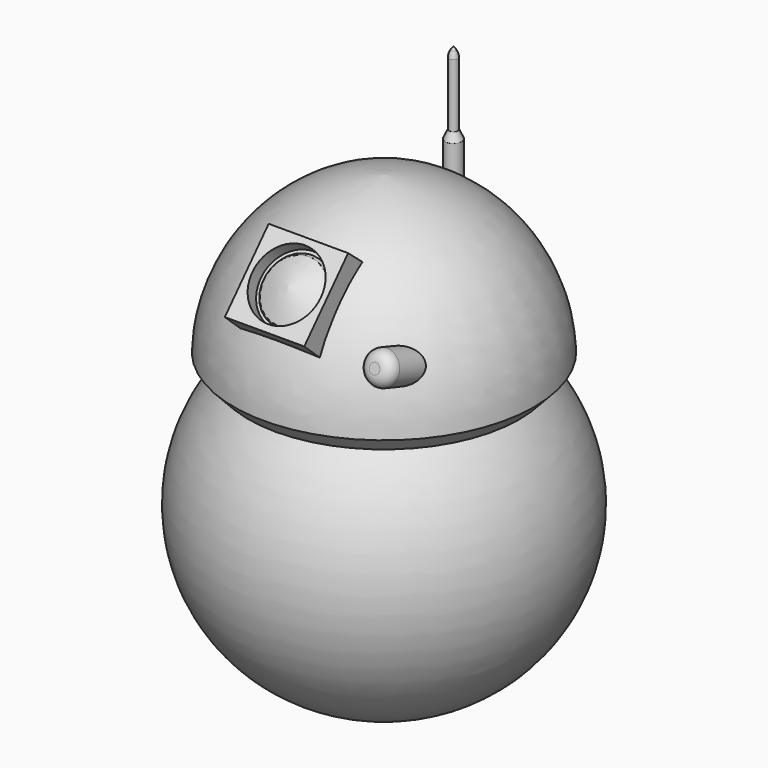
from build123d import *

# Parameters (mm, degrees)
F7_DEPTH = 18.288
F8_R     = 15.7921684899
F9_DEPTH = 6.604
F15_R    = 5.08
F16_R    = 5.08


with BuildPart() as f1:
    # F0 (on Front) → F1 (revolve)
    with BuildSketch(Plane.XZ):
        with BuildLine():
            Line((0, 77.0203024149), (0, -77.3050412536))
            ThreePointArc((0, -77.3050412536), (79.8093785121, -0.1423694193), (0, 77.0203024149))
        make_face()
    revolve(axis=Axis((0, 0, -0.1423694193), (0, 0, 1)))


with BuildPart() as f3:
    # F2 (on Front) → F3 (revolve)
    with BuildSketch(Plane.XZ):
        with BuildLine():
            Line((-69.1199526191, 61.6020485759), (-62.3490922153, 54.3798021972))
            ThreePointArc((-62.3490922153, 54.3798021972), (-33.4424698857, 72.8711770856), (0, 80.5604532361))
            Line((0, 80.5604532361), (0, 133.3731412888))
            ThreePointArc((0, 133.3731412888), (-48.2298855063, 110.6525536959), (-69.1199526191, 61.6020485759))
        make_face()
    revolve(axis=Axis((0, 0, 106.9667972624), (0, 0, 1)))


with BuildPart() as f5:
    # F4 (on Right) → F5 (revolve)
    with BuildSketch(Plane.YZ):
        with BuildLine():
            Line((-37.6473630313, 117.5783574581), (-43.1099124253, 117.5783574581))
            add(Edge.make_bspline(
                [(-43.1099124253, 117.5783574581), (-45.6695191469, 116.4036462387), (-50.3685346331, 114.2470703222), (-54.3983321793, 110.6990953442), (-55.3145445883, 110.0981011987)],
                knots=[0, 0, 0, 0, 0.4632741416, 0.8504948621, 0.8504948621, 0.8504948621, 0.8504948621], degree=3))
            Line((-55.3145445883, 110.0981011987), (-49.0153767169, 104.5863330364))
            Line((-49.0153767169, 104.5863330364), (-37.6473630313, 117.5783574581))
        make_face()
    revolve(axis=Axis((0, -52.1649606526, 107.3422171175), (0, 0.7525769153, -0.6585043558)))


with BuildPart() as f7:
    # F6 (on Right) → F7 (new body, symmetric)
    with BuildSketch(Plane.YZ):
        Polygon((-59.645216912, 89.2321169376), (-34.054864198, 117.1846613288), (-43.5066700909, 125.1279643094), (-68.7435230148, 97.561550531), align=None)
    extrude(amount=F7_DEPTH, both=True)


with BuildPart() as f9_tool:
    # F8 (on face) → F9 (new body)
    with BuildSketch(Plane(origin=(0, -85.9899317235, 78.7231620803), x_dir=(1, 0, 0), z_dir=(0, -0.7375852753, 0.6752539979))):
        with Locations((0, 44.3651229143)):
            Circle(F8_R)
    extrude(amount=-F9_DEPTH)


with BuildPart() as f3_1:
    add(f3.part)

    # F9: cut by f9_tool
    add(f9_tool.part, mode=Mode.SUBTRACT)


with BuildPart() as f7_1:
    add(f7.part)

    # F9: cut by f9_tool
    add(f9_tool.part, mode=Mode.SUBTRACT)


with BuildPart() as f11:
    # F10 (on Right) → F11 (revolve)
    with BuildSketch(Plane.YZ):
        Polygon((39.9532988667, 106.1036959291), (43.7825210392, 106.1036959291), (43.7825210392, 131.6318511963), (41.9955514371, 135.4610621929), (41.9955514371, 166.3501262665), (39.9532988667, 169.1582202911), align=None)
    revolve(axis=Axis((0, 39.9532988667, 137.6309581101), (0, 0, -1)))

    # F16
    f16_edges = [f11.edges().sort_by_distance(p)[0] for p in [
        (0, 37.911046, 166.350126),
    ]]
    fillet(f16_edges, radius=F16_R)


with BuildPart() as f14:
    # F13 (on offset) → F14 (revolve)
    with BuildSketch(Plane.YZ.offset(42.926)):
        Polygon((-35.6930941343, 84.8216339946), (-35.6930941343, 92.6510840654), (-56.6944193071, 99.6898593327), (-59.0535255471, 92.6510840654), align=None)
    revolve(axis=Axis((42.926, -47.3733098407, 88.73635903), (0, 0.9481628173, -0.3177849461)))

    # F15
    f15_edges = [f14.edges().sort_by_distance(p)[0] for p in [
        (42.926, -61.412632, 85.612309),
    ]]
    fillet(f15_edges, radius=F15_R)


solid = Compound([f1.part, f5.part, f3_1.part, f7_1.part, f11.part, f14.part])
